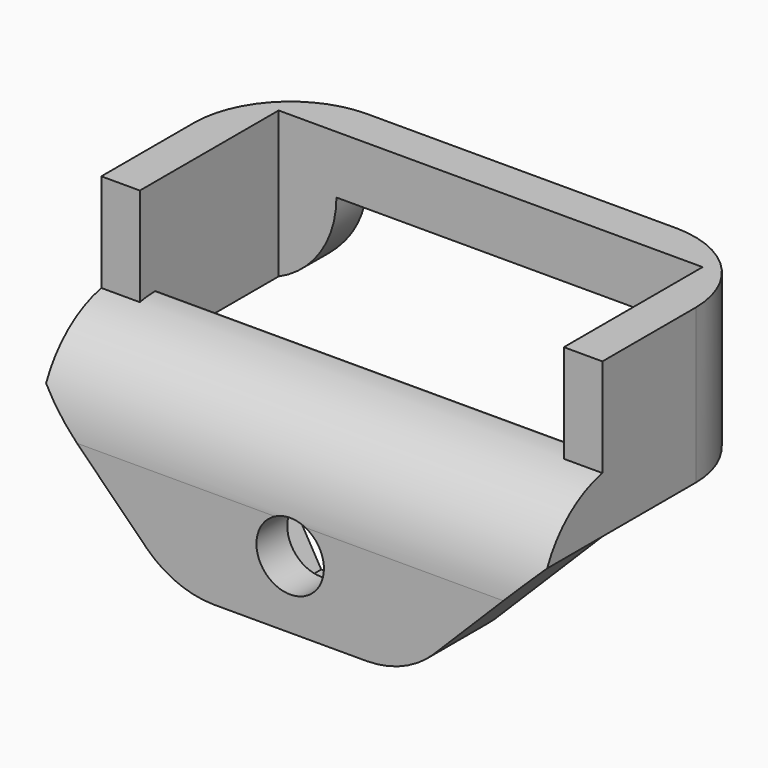
from build123d import *

# Parameters (mm, degrees)
F1_DEPTH      = 8
F2_DEPTH      = 3
F3_W          = 16
F3_H          = 5
F4_DEPTH      = 2
F5_DEPTH      = 7
F6_SIZE       = 7
F7_R          = 1.75
F8_DEPTH      = 4.001
F9_DEPTH      = 2
F10_T4_DEPTH  = 27
F10_T9_DEPTH  = 27
F11_T1_DEPTH  = 33.0048285071
F11_T3_DEPTH  = 14.359481388
F11_T8_DEPTH  = 51.0048285071
F11_T13_DEPTH = 51.0048285071


# Not quite as in the source:
# - a fillet or chamfer that OpenCascade refuses, or shapes differently, is made with other operations: its cross-section is extruded or revolved along the edge and cut away or added


with BuildPart() as f1:
    # F0 (on Top) → F1 (new body)
    with BuildSketch(Plane.XY):
        Polygon((13, -3.5), (13, 7.5), (-13, 7.5), (-13, -3.5), (-11, -3.5), (-11, -2.5), (-11, 5.5), (11, 5.5), (11, -2.5), (11, -3.5), align=None)
    extrude(amount=F1_DEPTH)

    # F0 (on Top) → F2 (join)
    with BuildSketch(Plane.XY):
        Polygon((7.5, -3.5), (11, -3.5), (11, -2.5), (-11, -2.5), (-11, -3.5), (-7.5, -3.5), align=None)
        Polygon((13, -7.5), (13, -3.5), (11, -3.5), (7.5, -3.5), (-7.5, -3.5), (-11, -3.5), (-13, -3.5), (-13, -7.5), (-11, -7.5), (-7.5, -7.5), (7.5, -7.5), (11, -7.5), align=None)
    extrude(amount=F2_DEPTH)

    # F3 (on face) → F4 (cut, through all)
    with BuildSketch(Plane(origin=(0, 7.5, 0), x_dir=(-1, 0, 0), z_dir=(0, 1, 0))):
        with Locations((0, 2.5)):
            Rectangle(F3_W, F3_H)
    extrude(amount=-F4_DEPTH, mode=Mode.SUBTRACT)

    # F0 (on Top) → F5 (join)
    with BuildSketch(Plane.XY):
        Polygon((13, -7.5), (13, -3.5), (11, -3.5), (7.5, -3.5), (-7.5, -3.5), (-11, -3.5), (-13, -3.5), (-13, -7.5), (-11, -7.5), (-7.5, -7.5), (7.5, -7.5), (11, -7.5), align=None)
    extrude(amount=-F5_DEPTH)

    # F6
    f6_edges = [f1.edges().sort_by_distance(p)[0] for p in [
        (13, -5.5, -7),
        (-13, -5.5, -7),
    ]]
    chamfer(f6_edges, length=F6_SIZE)

    # F7 (on face) → F8 (cut, through all)
    with BuildSketch(Plane(origin=(0, -3.5, 0), x_dir=(-1, 0, 0), z_dir=(0, 1, 0))):
        with Locations((0, -3.5)):
            Circle(F7_R)
    extrude(amount=-F8_DEPTH, mode=Mode.SUBTRACT)

    # F7 (on face) → F9 (cut)
    with BuildSketch(Plane(origin=(0, -3.5, 0), x_dir=(-1, 0, 0), z_dir=(0, 1, 0))):
        Polygon((1.5877132403, -6.25), (3.1754264805, -3.5), (1.5877132403, -0.75), (-1.5877132403, -0.75), (-3.1754264805, -3.5), (-1.5877132403, -6.25), align=None)
        with Locations((0, -3.5)):
            Circle(F7_R, mode=Mode.SUBTRACT)
    extrude(amount=-F9_DEPTH, mode=Mode.SUBTRACT)

    # F10: fillet of radius 5 on 2 edges, made by hand


with BuildPart() as f10_tool2:
    # F10_s3 → F10_t4 (new body)
    with BuildSketch(Plane.XZ.offset(-20)):
        with BuildLine():
            ThreePointArc((13, 0), (9.4644660941, 1.4644660941), (8, 5))
            Line((8, 5), (8, 0))
            Line((8, 0), (13, 0))
        make_face()
    extrude(amount=F10_T4_DEPTH)

    split(bisect_by=Plane.XZ.offset(2.5), keep=Keep.BOTTOM)


with BuildPart() as f1_1:
    add(f1.part)

    # F10_t1: cut F10_tool2
    add(f10_tool2.part, mode=Mode.SUBTRACT)


with BuildPart() as f10_tool7:
    # F10_s8 → F10_t9 (new body)
    with BuildSketch(Plane.XZ.offset(-20)):
        with BuildLine():
            ThreePointArc((-13, 0), (-9.4644660941, 1.4644660941), (-8, 5))
            Line((-8, 5), (-8, 0))
            Line((-8, 0), (-13, 0))
        make_face()
    extrude(amount=F10_T9_DEPTH)

    split(bisect_by=Plane.XZ.offset(2.5), keep=Keep.BOTTOM)


with BuildPart() as f1_2:
    add(f1_1.part)

    # F10_t6: cut F10_tool7
    add(f10_tool7.part, mode=Mode.SUBTRACT)

    # F11: fillet of radius 5 on 5 edges, made by hand

    # F11_s2 → F11_t1 (cut)
    with BuildSketch(Plane.XY.offset(-12.5024142536)):
        with BuildLine():
            ThreePointArc((-13.0004, 2.4990343146), (-11.5355339059, 6.0355339059), (-7.9990343146, 7.5004))
            Line((-7.9990343146, 7.5004), (-7.9990343146, 8.0005365685))
            ThreePointArc((-7.9990343146, 8.0005365685), (-10.4995171573, 8.0001365685), (-13, 8.0001365685))
            Line((-13, 8.0001365685), (-13.5001365685, 7.5))
            ThreePointArc((-13.5001365685, 7.5), (-13.5001365685, 4.9995171573), (-13.5005365685, 2.4990343146))
            Line((-13.5005365685, 2.4990343146), (-13.0004, 2.4990343146))
        make_face()
        with BuildLine():
            ThreePointArc((13.0004, 2.4990343146), (11.5355339059, 6.0355339059), (7.9990343146, 7.5004))
            Line((7.9990343146, 7.5004), (7.9990343146, 8.0005365685))
            ThreePointArc((7.9990343146, 8.0005365685), (10.4995171573, 8.0001365685), (13, 8.0001365685))
            Line((13, 8.0001365685), (13.5001365685, 7.5))
            ThreePointArc((13.5001365685, 7.5), (13.5001365685, 4.9995171573), (13.5005365685, 2.4990343146))
            Line((13.5005365685, 2.4990343146), (13.0004, 2.4990343146))
        make_face()
    extrude(amount=F11_T1_DEPTH, mode=Mode.SUBTRACT)

    # F11_s4 → F11_t3 (cut)
    with BuildSketch(Plane.XZ.offset(-1.679740694)):
        with BuildLine():
            ThreePointArc((3.928103761, -7.0004), (5.8424393631, -6.6196149734), (7.4653347232, -5.5352309622))
            Line((7.4653347232, -5.5352309622), (7.8190578194, -5.8889540584))
            ThreePointArc((7.8190578194, -5.8889540584), (7.0862490365, -6.621197156), (6.3537230962, -7.3537230962))
            Line((6.3537230962, -7.3537230962), (6, -7.50024))
            ThreePointArc((6, -7.50024), (4.9640518805, -7.50024), (3.928103761, -7.50064))
            Line((3.928103761, -7.50064), (3.928103761, -7.0004))
        make_face()
        with BuildLine():
            ThreePointArc((-7.4653347232, -5.5352309622), (-5.8424393631, -6.6196149734), (-3.928103761, -7.0004))
            Line((-3.928103761, -7.0004), (-3.928103761, -7.50064))
            ThreePointArc((-3.928103761, -7.50064), (-4.9640518805, -7.50024), (-6, -7.50024))
            Line((-6, -7.50024), (-6.3537230962, -7.3537230962))
            ThreePointArc((-6.3537230962, -7.3537230962), (-7.0862490365, -6.621197156), (-7.8190578194, -5.8889540584))
            Line((-7.8190578194, -5.8889540584), (-7.4653347232, -5.5352309622))
        make_face()
    extrude(amount=F11_T3_DEPTH, mode=Mode.SUBTRACT)


with BuildPart() as f11_tool6:
    # F11_s7 → F11_t8 (new body)
    with BuildSketch(Plane.YZ.offset(-25.5024142536)):
        with BuildLine():
            ThreePointArc((-2.4990343146, 3.0004), (-6.0355339059, 1.5355339059), (-7.5004, -2.0009656854))
            Line((-7.5004, -2.0009656854), (-8.0005365685, -2.0009656854))
            ThreePointArc((-8.0005365685, -2.0009656854), (-8.0001365685, 0.4995171573), (-8.0001365685, 3))
            Line((-8.0001365685, 3), (-7.5, 3.5001365685))
            ThreePointArc((-7.5, 3.5001365685), (-4.9995171573, 3.5001365685), (-2.4990343146, 3.5005365685))
            Line((-2.4990343146, 3.5005365685), (-2.4990343146, 3.0004))
        make_face()
    extrude(amount=F11_T8_DEPTH)

    split(bisect_by=Plane.XZ.offset(3.5), keep=Keep.TOP)


with BuildPart() as f1_3:
    add(f1_2.part)

    # F11_t5: cut F11_tool6
    add(f11_tool6.part, mode=Mode.SUBTRACT)


with BuildPart() as f11_tool11:
    # F11_s12 → F11_t13 (new body)
    with BuildSketch(Plane.YZ.offset(-25.5024142536)):
        with BuildLine():
            ThreePointArc((-2.4990343146, 3.0004), (-6.0355339059, 1.5355339059), (-7.5004, -2.0009656854))
            Line((-7.5004, -2.0009656854), (-8.0005365685, -2.0009656854))
            ThreePointArc((-8.0005365685, -2.0009656854), (-8.0001365685, 0.4995171573), (-8.0001365685, 3))
            Line((-8.0001365685, 3), (-7.5, 3.5001365685))
            ThreePointArc((-7.5, 3.5001365685), (-4.9995171573, 3.5001365685), (-2.4990343146, 3.5005365685))
            Line((-2.4990343146, 3.5005365685), (-2.4990343146, 3.0004))
        make_face()
    extrude(amount=F11_T13_DEPTH)

    split(bisect_by=Plane.YZ.offset(11), keep=Keep.BOTTOM)

    split(bisect_by=Plane.YZ.offset(-11), keep=Keep.TOP)


with BuildPart() as f1_4:
    add(f1_3.part)

    # F11_t10: cut F11_tool11
    add(f11_tool11.part, mode=Mode.SUBTRACT)


solid = f1_4.part
